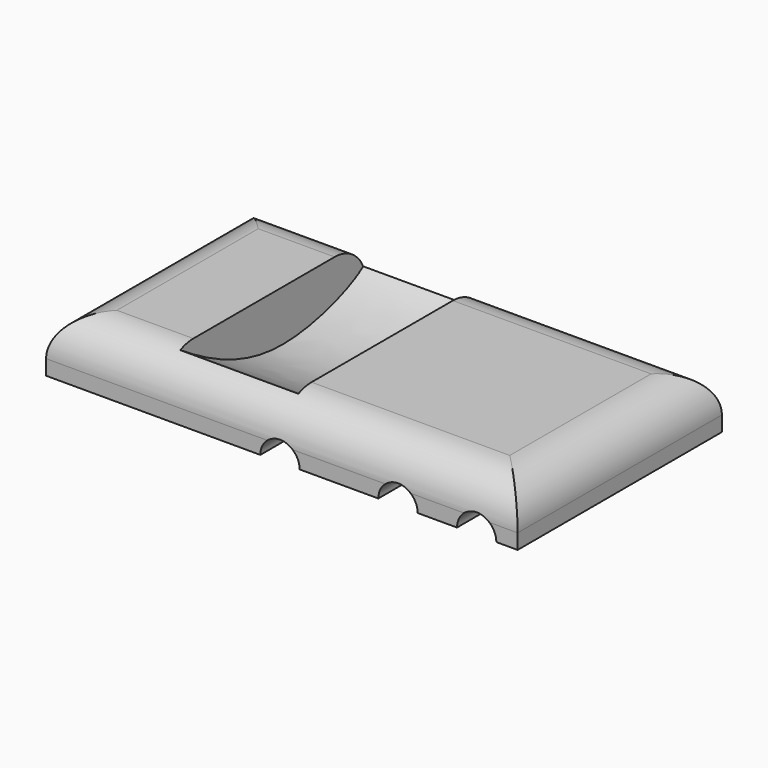
from build123d import *

# Parameters (mm, degrees)
F0_W        = 304.4815510511
F0_H        = 164.8949235678
F1_DEPTH    = 35.13393
F3_DEPTH    = 76.30524
F4_R        = 12.7
F5_DEPTH    = 164.8959236678
F6_T1_DEPTH = 291.8949235678
F6_T3_DEPTH = 431.4815510511


# Not quite as in the source:
# - a fillet or chamfer that OpenCascade refuses, or shapes differently, is made with other operations: its cross-section is extruded or revolved along the edge and cut away or added


with BuildPart() as f1:
    # F0 (on Top) → F1 (new body)
    with BuildSketch(Plane.XY):
        with Locations((1.1980161071, -3.480002284)):
            Rectangle(F0_W, F0_H)
    extrude(amount=F1_DEPTH)

    # F2 (on Right) → F3 (cut)
    with BuildSketch(Plane.YZ):
        with BuildLine():
            add(Edge.make_bspline(
                [(-153.2041430473, 84.2628479004), (-91.991528101, 80.6964321278), (-18.1249389438, 101.4390649478), (-6.3535316821, 35.464664407), (123.7363166686, 35.8483556733), (-7.6536515228, -20.5708818303), (-72.9342844873, 34.9796073045), (-103.3804491162, 54.5991994441)],
                knots=[0, 0, 0, 0, 0.2418010288, 0.3897431708, 0.5754176067, 0.7622533627, 1, 1, 1, 1], degree=3))
            add(Edge.make_bspline(
                [(-153.2041430473, 84.2628479004), (-136.2230330706, 76.9635861119), (-120.361559093, 61.8984612326), (-103.3804491162, 54.5991994441)],
                knots=[0, 0, 0, 0, 57.985623362, 57.985623362, 57.985623362, 57.985623362], degree=3))
        make_face()
    extrude(amount=-F3_DEPTH, mode=Mode.SUBTRACT)

    # F4 (on face) → F5 (cut, through all)
    with BuildSketch(Plane(origin=(0, 78.9674594998, 0), x_dir=(-1, 0, 0), z_dir=(0, 1, 0))):
        with Locations((-127, 0)):
            Circle(F4_R)
        with Locations((-76.2, 0)):
            Circle(F4_R)
        Circle(F4_R)
    extrude(amount=-F5_DEPTH, mode=Mode.SUBTRACT)

    # F6: fillet of radius 25.4 on 4 edges, made by hand

    # F6_s2 → F6_t1 (cut)
    with BuildSketch(Plane.XZ.offset(-142.4674594998)):
        with BuildLine():
            ThreePointArc((128.0387916327, 35.13393), (145.9993038748, 27.6944422421), (153.4387916327, 9.73393))
            Line((153.4387916327, 9.73393), (153.4387916327, 35.13393))
            Line((153.4387916327, 35.13393), (128.0387916327, 35.13393))
        make_face()
        with BuildLine():
            ThreePointArc((-151.0427594185, 9.73393), (-143.6032716606, 27.6944422421), (-125.6427594185, 35.13393))
            Line((-125.6427594185, 35.13393), (-151.0427594185, 35.13393))
            Line((-151.0427594185, 35.13393), (-151.0427594185, 9.73393))
        make_face()
    extrude(amount=F6_T1_DEPTH, mode=Mode.SUBTRACT)

    # F6_s4 → F6_t3 (cut)
    with BuildSketch(Plane.YZ.offset(-214.5427594185)):
        with BuildLine():
            ThreePointArc((78.9674594998, 9.73393), (71.527971742, 27.6944422421), (53.5674594998, 35.13393))
            Line((53.5674594998, 35.13393), (78.9674594998, 35.13393))
            Line((78.9674594998, 35.13393), (78.9674594998, 9.73393))
        make_face()
        with BuildLine():
            ThreePointArc((-60.5274640679, 35.13393), (-78.4879763101, 27.6944422421), (-85.9274640679, 9.73393))
            Line((-85.9274640679, 9.73393), (-85.9274640679, 35.13393))
            Line((-85.9274640679, 35.13393), (-60.5274640679, 35.13393))
        make_face()
    extrude(amount=F6_T3_DEPTH, mode=Mode.SUBTRACT)


solid = f1.part
